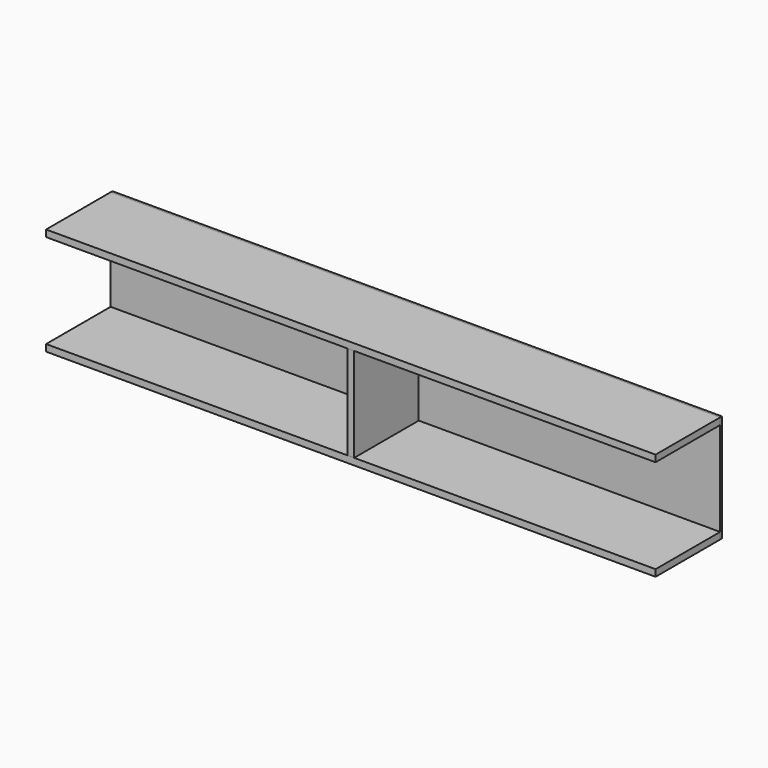
from build123d import *

# Parameters (mm, degrees)
F0_W          = 1727.2
F0_H          = 304.8
F1_DEPTH      = 6.35
F3_E1_0_W     = 1727.2
F3_E1_0_H     = 228.6
F4_DEPTH      = 19.05
F6_W          = 228.6
F6_H          = 266.7
F7_DEPTH      = 9.525
F7_DEPTH_BACK = 9.525


# Not quite as in the source:
# - a feature names something its author has since deleted; it is built from what else it names


with BuildPart() as f1:
    # F0 (on Front) → F1 (new body)
    with BuildSketch(Plane.XZ):
        Rectangle(F0_W, F0_H)
    extrude(amount=-F1_DEPTH)


with BuildPart() as f4:
    # F3_E1_0 (on explicit) → F4 (new body)
    with BuildSketch(Plane(origin=(863.6, 0, 152.4), x_dir=(-1, 0, 0), z_dir=(0, 0, 1))):
        with Locations((863.6, 114.3)):
            Rectangle(F3_E1_0_W, F3_E1_0_H)
    extrude(amount=-F4_DEPTH)


with BuildPart() as f5_1:
    # F5: instance of F4
    add(f4.part.mirror(Plane.XY))


with BuildPart() as f7:
    # F6 (on Right) → F7 (new body, two sides)
    with BuildSketch(Plane.YZ) as f7_sk:
        with Locations((-114.3, 0)):
            Rectangle(F6_W, F6_H)
    extrude(amount=F7_DEPTH)
    extrude(f7_sk.sketch, amount=-F7_DEPTH_BACK)


solid = Compound([f1.part, f4.part, f5_1.part, f7.part])
